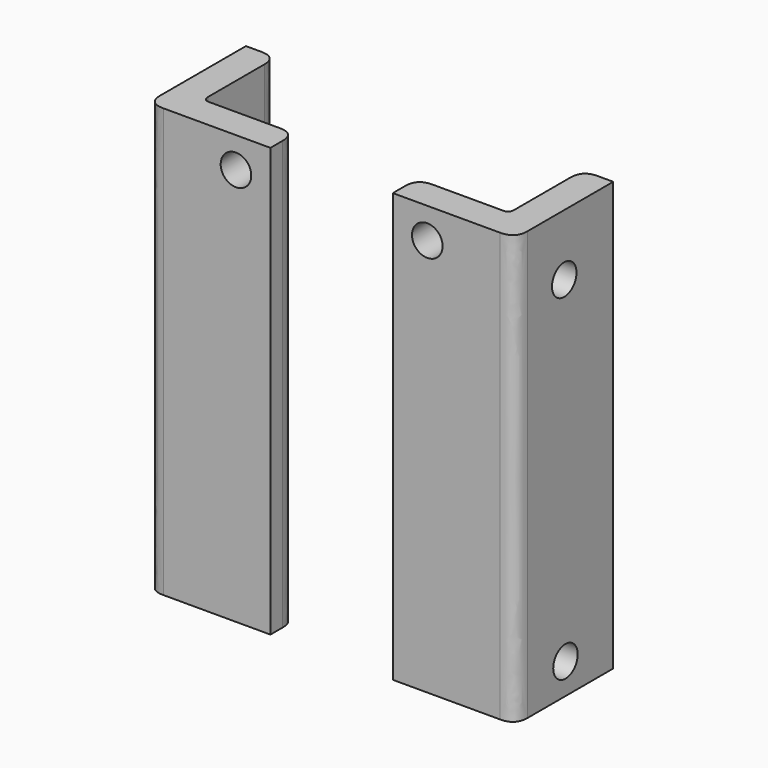
from build123d import *

# Parameters (mm, degrees)
F1_DEPTH      = 88.9
F2_T1_DEPTH   = 104.775
F3_T1_DEPTH   = 104.775
F5_DEPTH      = 88.9
F6_T1_DEPTH   = 104.775
F7_T1_DEPTH   = 88.9
F7_2_T1_DEPTH = 88.9
F8_T1_DEPTH   = 104.775
F10_R         = 3.175
F11_DEPTH     = 6.35
F9_R          = 3.175
F12_DEPTH     = 6.35
F14_R         = 3.175
F15_DEPTH     = 6.35
F13_R         = 3.175
F16_DEPTH     = 6.35
F17_R         = 3.175
F19_DEPTH     = 6.35
F18_R         = 3.175
F20_DEPTH     = 6.35


# Not quite as in the source:
# - a fillet or chamfer that OpenCascade refuses, or shapes differently, is made with other operations: its cross-section is extruded or revolved along the edge and cut away or added


with BuildPart() as f1:
    # F0 (on Top) → F1 (new body)
    with BuildSketch(Plane.XY):
        Polygon((-19.05, -11.4788501549), (-19.05, 7.5711498451), (-25.4, 7.5711498451), (-25.4, -17.8288501549), (0, -17.8288501549), (0, -11.4788501549), align=None)
    extrude(amount=F1_DEPTH)

    # F2: fillet of radius 3.175 on 2 edges, made by hand

    # F2_s2 → F2_t1 (cut)
    with BuildSketch(Plane.XY.offset(-7.9375)):
        with BuildLine():
            add(Edge.make_bspline(
                [(-19.05, 4.3961498451), (-19.05, 7.5711498451), (-22.225, 7.5711498451)],
                knots=[0, 0, 0, 1, 1, 1], degree=2, weights=[1, 1, 1]))
            Line((-22.225, 7.5711498451), (-19.05, 7.5711498451))
            Line((-19.05, 7.5711498451), (-19.05, 4.3961498451))
        make_face()
        with BuildLine():
            add(Edge.make_bspline(
                [(0, -14.6538501549), (0, -11.4788501549), (-3.175, -11.4788501549)],
                knots=[0, 0, 0, 1, 1, 1], degree=2, weights=[1, 1, 1]))
            Line((-3.175, -11.4788501549), (0, -11.4788501549))
            Line((0, -11.4788501549), (0, -14.6538501549))
        make_face()
    extrude(amount=F2_T1_DEPTH, mode=Mode.SUBTRACT)

    # F3: fillet of radius 3.175 on 1 edges, made by hand

    # F3_s2 → F3_t1 (cut)
    with BuildSketch(Plane.XY.offset(-7.9375)):
        with BuildLine():
            add(Edge.make_bspline(
                [(-22.225, -17.8288501549), (-25.4, -17.8288501549), (-25.4, -14.6538501549)],
                knots=[0, 0, 0, 1, 1, 1], degree=2, weights=[1, 1, 1]))
            Line((-25.4, -14.6538501549), (-25.4, -17.8288501549))
            Line((-25.4, -17.8288501549), (-22.225, -17.8288501549))
        make_face()
    extrude(amount=F3_T1_DEPTH, mode=Mode.SUBTRACT)

    # F7#2: fillet of radius 1.27 on 1 edges, made by hand

    # F7_2_s2 → F7_2_t1 (join)
    with BuildSketch(Plane.XY):
        with BuildLine():
            add(Edge.make_bspline(
                [(-19.05, -10.2088501549), (-19.05, -11.4788501549), (-17.78, -11.4788501549)],
                knots=[0, 0, 0, 1, 1, 1], degree=2, weights=[1, 1, 1]))
            Line((-17.78, -11.4788501549), (-19.05, -11.4788501549))
            Line((-19.05, -11.4788501549), (-19.05, -10.2088501549))
        make_face()
    extrude(amount=F7_2_T1_DEPTH)

    # F9 (on face) → F12 (cut)
    with BuildSketch(Plane.YZ.offset(-19.05)):
        with Locations((-4.8113501549, 6.35)):
            Circle(F9_R)
    extrude(amount=-F12_DEPTH, mode=Mode.SUBTRACT)

    # F14 (on face) → F15 (cut)
    with BuildSketch(Plane(origin=(-25.4, 0, 0), x_dir=(0, -1, 0), z_dir=(-1, 0, 0))):
        with Locations((5.1288501549, 76.2)):
            Circle(F14_R)
    extrude(amount=-F15_DEPTH, mode=Mode.SUBTRACT)

    # F18 (on face) → F20 (cut)
    with BuildSketch(Plane(origin=(0, -11.4788501549, 0), x_dir=(-1, 0, 0), z_dir=(0, 1, 0))):
        with Locations((7.14375, 82.55)):
            Circle(F18_R)
    extrude(amount=-F20_DEPTH, mode=Mode.SUBTRACT)


with BuildPart() as f5:
    # F4 (on Top) → F5 (new body)
    with BuildSketch(Plane.XY):
        Polygon((25.4, -11.4788501549), (25.4, -17.8288501549), (50.8, -17.8288501549), (50.8, 7.5711498451), (44.45, 7.5711498451), (44.45, -11.4788501549), align=None)
    extrude(amount=F5_DEPTH)

    # F6: fillet of radius 3.175 on 2 edges, made by hand

    # F6_s2 → F6_t1 (cut)
    with BuildSketch(Plane.XY.offset(-7.9375)):
        with BuildLine():
            add(Edge.make_bspline(
                [(25.4, -14.6538501549), (25.4, -11.4788501549), (28.575, -11.4788501549)],
                knots=[0, 0, 0, 1, 1, 1], degree=2, weights=[1, 1, 1]))
            Line((28.575, -11.4788501549), (25.4, -11.4788501549))
            Line((25.4, -11.4788501549), (25.4, -14.6538501549))
        make_face()
        with BuildLine():
            add(Edge.make_bspline(
                [(47.625, 7.5711498451), (44.45, 7.5711498451), (44.45, 4.3961498451)],
                knots=[0, 0, 0, 1, 1, 1], degree=2, weights=[1, 1, 1]))
            Line((44.45, 4.3961498451), (44.45, 7.5711498451))
            Line((44.45, 7.5711498451), (47.625, 7.5711498451))
        make_face()
    extrude(amount=F6_T1_DEPTH, mode=Mode.SUBTRACT)

    # F7: fillet of radius 1.27 on 1 edges, made by hand

    # F7_s2 → F7_t1 (join)
    with BuildSketch(Plane.XY):
        with BuildLine():
            add(Edge.make_bspline(
                [(43.18, -11.4788501549), (44.45, -11.4788501549), (44.45, -10.2088501549)],
                knots=[0, 0, 0, 1, 1, 1], degree=2, weights=[1, 1, 1]))
            Line((44.45, -10.2088501549), (44.45, -11.4788501549))
            Line((44.45, -11.4788501549), (43.18, -11.4788501549))
        make_face()
    extrude(amount=F7_T1_DEPTH)

    # F8: fillet of radius 3.175 on 1 edges, made by hand

    # F8_s2 → F8_t1 (cut)
    with BuildSketch(Plane.XY.offset(-7.9375)):
        with BuildLine():
            add(Edge.make_bspline(
                [(47.625, -17.8288501549), (50.8, -17.8288501549), (50.8, -14.6538501549)],
                knots=[0, 0, 0, 1, 1, 1], degree=2, weights=[1, 1, 1]))
            Line((50.8, -14.6538501549), (50.8, -17.8288501549))
            Line((50.8, -17.8288501549), (47.625, -17.8288501549))
        make_face()
    extrude(amount=F8_T1_DEPTH, mode=Mode.SUBTRACT)

    # F10 (on face) → F11 (cut)
    with BuildSketch(Plane(origin=(44.45, 0, 0), x_dir=(0, -1, 0), z_dir=(-1, 0, 0))):
        with Locations((4.8113501549, 6.35)):
            Circle(F10_R)
    extrude(amount=-F11_DEPTH, mode=Mode.SUBTRACT)

    # F13 (on face) → F16 (cut)
    with BuildSketch(Plane.YZ.offset(50.8)):
        with Locations((-5.1288501549, 76.2)):
            Circle(F13_R)
    extrude(amount=-F16_DEPTH, mode=Mode.SUBTRACT)

    # F17 (on face) → F19 (cut)
    with BuildSketch(Plane(origin=(0, -11.4788501549, 0), x_dir=(-1, 0, 0), z_dir=(0, 1, 0))):
        with Locations((-32.54375, 82.55)):
            Circle(F17_R)
    extrude(amount=-F19_DEPTH, mode=Mode.SUBTRACT)


solid = Compound([f1.part, f5.part])
